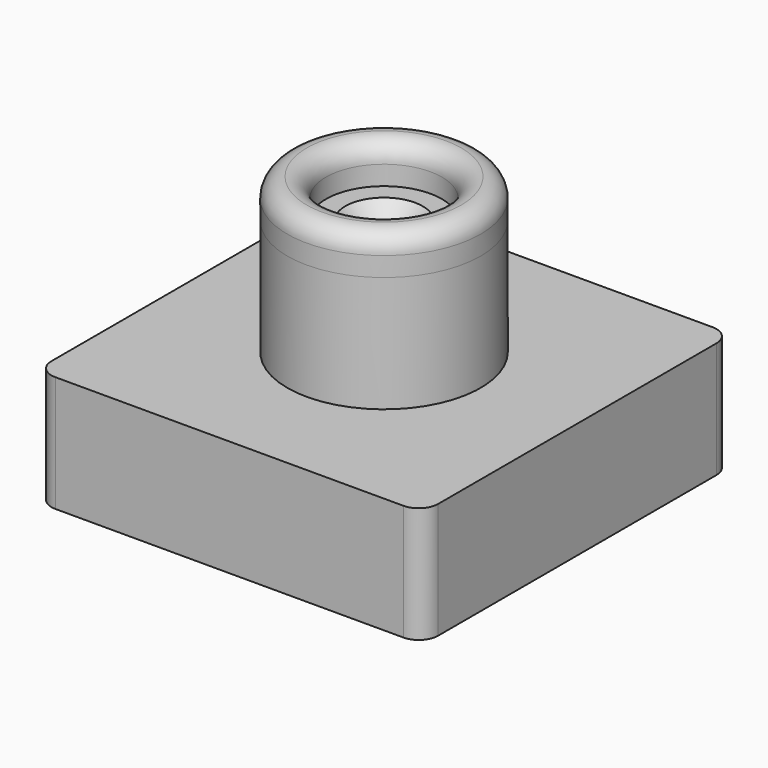
from build123d import *

# Parameters (mm, degrees)
F1_DEPTH       = 50
F0_W           = 25
F0_H           = 30
F4_D           = 10
F4_CSINK_D     = 20
F4_CSINK_ANGLE = 90
F5_R           = 5
F3_R           = 25
F3_R_2         = 15
F6_DEPTH       = 10
F7_R           = 4.99999


# Not quite as in the source:
# - a fillet or chamfer is up to 0.001 mm smaller than in the source, because OpenCascade refuses the exact size


with BuildPart() as f1:
    # F0 (on Front) → F1 (new body, symmetric)
    with BuildSketch(Plane.XZ):
        Polygon((50, 15), (25, 15), (0, 15), (0, -15), (50, -15), align=None)
        Polygon((0, -15), (0, 15), (-25, 15), (-50, 15), (-50, -15), align=None)
    extrude(amount=F1_DEPTH, both=True)

    # F0 (on Front) → F2 (revolve)
    with BuildSketch(Plane.XZ):
        with Locations((-12.5, 30)):
            Rectangle(F0_W, F0_H)
    revolve(axis=Axis((0, 0, 15), (0, 0, -1)))

    # F4 (through all)
    with Locations(Plane.XY.offset(45)):
        with Locations((0, 0)):
            CounterSinkHole(F4_D / 2, F4_CSINK_D / 2, counter_sink_angle=F4_CSINK_ANGLE)

    # F5
    f5_edges = [f1.edges().sort_by_distance(p)[0] for p in [
        (-50, 50, 0),
        (50, 50, 0),
        (50, -50, 0),
        (-50, -50, 0),
    ]]
    fillet(f5_edges, radius=F5_R)

    # F3 (on face) → F6 (join)
    with BuildSketch(Plane.XY.offset(45)):
        Circle(F3_R)
        Circle(F3_R_2, mode=Mode.SUBTRACT)
    extrude(amount=F6_DEPTH)

    # F7 (radius 5 in the source; OpenCascade refuses exactly that, so slightly less here)
    f7_edges = [f1.edges().sort_by_distance(p)[0] for p in [
        (-25, 0, 55),
        (-25, 0, 30),
        (-15, 0, 55),
    ]]
    fillet(f7_edges, radius=F7_R)


solid = f1.part
